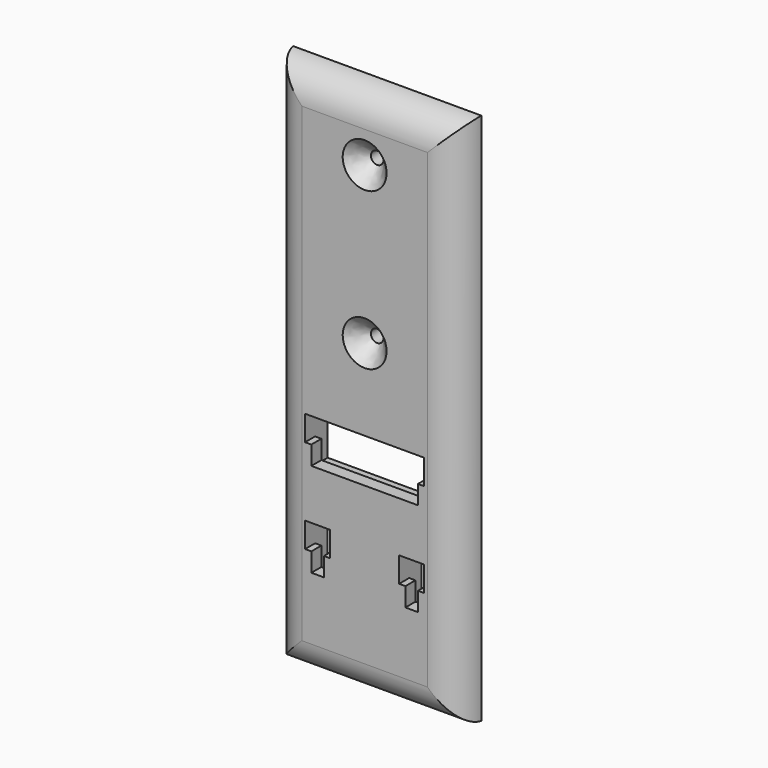
from build123d import *
from build123d import SkipClean  # not in build123d's __all__

# Parameters (mm, degrees)
F0_R        = 2
F1_DEPTH    = 5
F0_W        = 22
F0_H        = 2
F0_W_2      = 2
F0_H_2      = 6
F0_W_3      = 4
F2_DEPTH    = 4
F3_SIZE     = 5
F4_T1_DEPTH = 219.7493718553
F4_T3_DEPTH = 109.7493718553


# Not quite as in the source:
# - a fillet or chamfer that OpenCascade refuses, or shapes differently, is made with other operations: its cross-section is extruded or revolved along the edge and cut away or added
# - a feature names something its author has since deleted; it is built from what else it names


with BuildPart() as f1:
    # F0 (on Front) → F1 (new body)
    with BuildSketch(Plane.XZ):
        with BuildLine():
            Line((-30, 150), (-30, 80))
            Line((-30, 80), (-2, 80))
            ThreePointArc((-2, 80), (0, 82), (2, 80))
            Line((2, 80), (30, 80))
            Line((30, 80), (30, 150))
            Line((30, 150), (-30, 150))
        make_face()
        with Locations((0, 130)):
            Circle(F0_R, mode=Mode.SUBTRACT)
        with BuildLine():
            Line((-30, 0), (0, 0))
            Line((0, 0), (30, 0))
            Line((30, 0), (30, 80))
            Line((30, 80), (2, 80))
            ThreePointArc((2, 80), (0, 78), (-2, 80))
            Line((-2, 80), (-30, 80))
            Line((-30, 80), (-30, 0))
        make_face()
        Polygon((-11, 24), (-11, 16), (-11, 10), (-11, 8), (-13, 8), (-17, 8), (-19, 8), (-19, 10), (-19, 16), (-19, 24), align=None, mode=Mode.SUBTRACT)
        Polygon((19, 24), (19, 16), (19, 10), (19, 8), (17, 8), (13, 8), (11, 8), (11, 10), (11, 16), (11, 24), align=None, mode=Mode.SUBTRACT)
        Polygon((-19, 54), (-11, 54), (11, 54), (19, 54), (19, 46), (19, 40), (19, 38), (17, 38), (13, 38), (11, 38), (-11, 38), (-13, 38), (-17, 38), (-19, 38), (-19, 40), (-19, 46), (-19, 48), align=None, mode=Mode.SUBTRACT)
        Polygon((30, 0), (0, 0), (-30, 0), (-30, -20), (30, -20), align=None)
    extrude(amount=-F1_DEPTH)

    # F0 (on Front) → F2 (join)
    with BuildSketch(Plane.XZ):
        with BuildLine():
            Line((-30, 0), (0, 0))
            Line((0, 0), (30, 0))
            Line((30, 0), (30, 80))
            Line((30, 80), (2, 80))
            ThreePointArc((2, 80), (0, 78), (-2, 80))
            Line((-2, 80), (-30, 80))
            Line((-30, 80), (-30, 0))
        make_face()
        Polygon((-11, 24), (-11, 16), (-11, 10), (-11, 8), (-13, 8), (-17, 8), (-19, 8), (-19, 10), (-19, 16), (-19, 24), align=None, mode=Mode.SUBTRACT)
        Polygon((19, 24), (19, 16), (19, 10), (19, 8), (17, 8), (13, 8), (11, 8), (11, 10), (11, 16), (11, 24), align=None, mode=Mode.SUBTRACT)
        Polygon((-19, 54), (-11, 54), (11, 54), (19, 54), (19, 46), (19, 40), (19, 38), (17, 38), (13, 38), (11, 38), (-11, 38), (-13, 38), (-17, 38), (-19, 38), (-19, 40), (-19, 46), (-19, 48), align=None, mode=Mode.SUBTRACT)
        with BuildLine():
            Line((-30, 150), (-30, 80))
            Line((-30, 80), (-2, 80))
            ThreePointArc((-2, 80), (0, 82), (2, 80))
            Line((2, 80), (30, 80))
            Line((30, 80), (30, 150))
            Line((30, 150), (-30, 150))
        make_face()
        with Locations((0, 130)):
            Circle(F0_R, mode=Mode.SUBTRACT)
        Polygon((30, 0), (0, 0), (-30, 0), (-30, -20), (30, -20), align=None)
        with Locations((0, 39)):
            Rectangle(F0_W, F0_H)
        with Locations((-18, 43)):
            Rectangle(F0_W_2, F0_H_2)
        with Locations((18, 43)):
            Rectangle(F0_W_2, F0_H_2)
        with Locations((-18, 13)):
            Rectangle(F0_W_2, F0_H_2)
        with Locations((-12, 13)):
            Rectangle(F0_W_2, F0_H_2)
        with Locations((12, 13)):
            Rectangle(F0_W_2, F0_H_2)
        with Locations((18, 13)):
            Rectangle(F0_W_2, F0_H_2)
        with Locations((-15, 39)):
            Rectangle(F0_W_3, F0_H)
        with Locations((15, 39)):
            Rectangle(F0_W_3, F0_H)
        with Locations((-15, 9)):
            Rectangle(F0_W_3, F0_H)
        with Locations((15, 9)):
            Rectangle(F0_W_3, F0_H)
        with Locations((-18, 39)):
            Rectangle(F0_W_2, F0_H)
        with Locations((-12, 39)):
            Rectangle(F0_W_2, F0_H)
        with Locations((12, 39)):
            Rectangle(F0_W_2, F0_H)
        with Locations((18, 39)):
            Rectangle(F0_W_2, F0_H)
        with Locations((-18, 9)):
            Rectangle(F0_W_2, F0_H)
        with Locations((-12, 9)):
            Rectangle(F0_W_2, F0_H)
        with Locations((12, 9)):
            Rectangle(F0_W_2, F0_H)
        with Locations((18, 9)):
            Rectangle(F0_W_2, F0_H)
    with SkipClean():  # cleaning this boolean's faces spoils the solid; the shape is the same uncleaned
        extrude(amount=F2_DEPTH)

    # F3
    f3_edges = [f1.edges().sort_by_distance(p)[0] for p in [
        (-2, -4, 130),
        (2, -4, 80),
    ]]
    chamfer(f3_edges, length=F3_SIZE)

    # F4: fillet of radius 10 on 4 edges, made by hand

    # F4_s2 → F4_t1 (cut)
    with BuildSketch(Plane.XY.offset(-44.8746859277)):
        with BuildLine():
            ThreePointArc((-20.0501256289, -4), (-26.7583295614, -1.4161984871), (-30, 5))
            Line((-30, 5), (-30, -4))
            Line((-30, -4), (-20.0501256289, -4))
        make_face()
        with BuildLine():
            ThreePointArc((20.0501256289, -4), (26.7583295614, -1.4161984871), (30, 5))
            Line((30, 5), (30, -4))
            Line((30, -4), (20.0501256289, -4))
        make_face()
    extrude(amount=F4_T1_DEPTH, mode=Mode.SUBTRACT)

    # F4_s4 → F4_t3 (cut)
    with BuildSketch(Plane.YZ.offset(-54.8746859277)):
        with BuildLine():
            ThreePointArc((-4, 140.0501256289), (-1.4161984871, 146.7583295614), (5, 150))
            Line((5, 150), (-4, 150))
            Line((-4, 150), (-4, 140.0501256289))
        make_face()
        with BuildLine():
            ThreePointArc((-4, -10.0501256289), (-1.4161984871, -16.7583295614), (5, -20))
            Line((5, -20), (-4, -20))
            Line((-4, -20), (-4, -10.0501256289))
        make_face()
    extrude(amount=F4_T3_DEPTH, mode=Mode.SUBTRACT)


solid = f1.part
